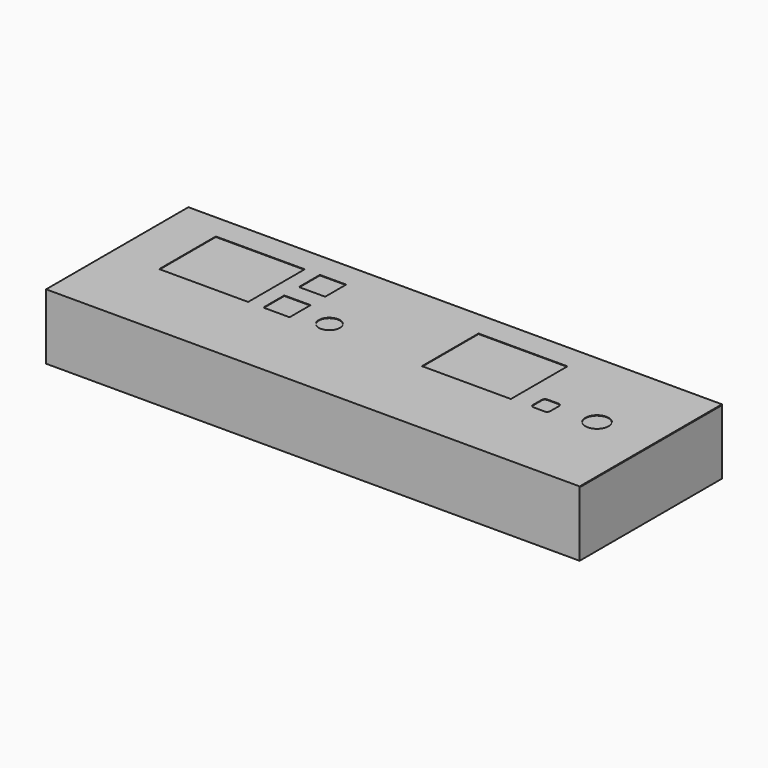
from build123d import *

# Parameters (mm, degrees)
F1_DEPTH = 209.55
F2_W     = 20.6375
F2_H     = 20.6375
F3_DEPTH = 0.4064


# Not quite as in the source:
# - the dataset's text gives a spline's control points without its knots; the knots are read off the source's solid


with BuildPart() as f1:
    # F0 (on Right) → F1 (new body, symmetric)
    with BuildSketch(Plane.YZ):
        Polygon((-139.7, 0), (0, 0), (0, 50.8), (-139.2936, 50.8), (-139.2936, 51.054), (0, 51.054), (0, 51.4604), (-139.7, 51.4604), align=None)
    extrude(amount=F1_DEPTH, both=True)

    # F2 (on face) → F3 (cut, through all)
    with BuildSketch(Plane.XY.offset(51.4604)):
        with BuildLine():
            add(Edge.make_bspline(
                [(120.2687199611, -62.5889714683), (119.8277505611, -63.0292296683), (119.5707533611, -63.6493706683), (119.5707533611, -64.2722294683)],
                knots=[1, 1, 1, 1, 2, 2, 2, 2], degree=3))
            Line((119.5707533611, -64.2722294683), (119.5707533611, -73.0035048683))
            add(Edge.make_bspline(
                [(119.5707533611, -73.0035048683), (119.5707533611, -73.6270748683), (119.8277505611, -74.2471650683), (120.2687199611, -74.6874486683)],
                knots=[0, 0, 0, 0, 1, 1, 1, 1], degree=3))
            add(Edge.make_bspline(
                [(120.2687199611, -74.6874486683), (120.7090289611, -75.1284180683), (121.3291445611, -75.3847548683), (121.9520033611, -75.3847548683)],
                knots=[1, 1, 1, 1, 2, 2, 2, 2], degree=3))
            Line((121.9520033611, -75.3847548683), (130.6832533611, -75.3847548683))
            add(Edge.make_bspline(
                [(130.6832533611, -75.3847548683), (131.3068233611, -75.3847548683), (131.9269389611, -75.1284180683), (132.3671971611, -74.6874486683)],
                knots=[0, 0, 0, 0, 1, 1, 1, 1], degree=3))
            add(Edge.make_bspline(
                [(132.3671971611, -74.6874486683), (132.8081665611, -74.2471650683), (133.0645033611, -73.6270748683), (133.0645033611, -73.0035048683)],
                knots=[1, 1, 1, 1, 2, 2, 2, 2], degree=3))
            Line((133.0645033611, -73.0035048683), (133.0645033611, -64.2722294683))
            add(Edge.make_bspline(
                [(133.0645033611, -64.2722294683), (133.0645033611, -63.6493706683), (132.8081665611, -63.0292296683), (132.3671971611, -62.5889714683)],
                knots=[0, 0, 0, 0, 1, 1, 1, 1], degree=3))
            add(Edge.make_bspline(
                [(132.3671971611, -62.5889714683), (131.9269389611, -62.1480020683), (131.3068233611, -61.8909794683), (130.6832533611, -61.8909794683)],
                knots=[1, 1, 1, 1, 2, 2, 2, 2], degree=3))
            Line((130.6832533611, -61.8909794683), (121.9520033611, -61.8909794683))
            add(Edge.make_bspline(
                [(121.9520033611, -61.8909794683), (121.3291445611, -61.8909794683), (120.7090289611, -62.1480020683), (120.2687199611, -62.5889714683)],
                knots=[0, 0, 0, 0, 1, 1, 1, 1], degree=3))
        make_face()
        Polygon((-172.1320160389, -19.8222294683), (-172.1320160389, -75.3847548683), (-102.2820160389, -75.3847548683), (-102.2821938389, -19.8222294683), align=None)
        Polygon((-90.3757660389, -75.3847548683), (-69.7382660389, -75.3847548683), (-69.7384438389, -54.7472294683), (-90.3759438389, -54.7472294683), align=None)
        with Locations((-80.0571938389, -30.1409794683)):
            Rectangle(F2_W, F2_H)
        Polygon((34.2429839611, -75.3847548683), (104.0926283611, -75.3847548683), (104.0926283611, -19.8222294683), (34.2426283611, -19.8222294683), align=None)
        with BuildLine():
            add(Edge.make_bspline(
                [(-39.2385048389, -61.1578846683), (-40.7817326389, -59.6144790683), (-42.9500798389, -58.7159794683), (-45.1321938389, -58.7159794683)],
                knots=[7, 7, 7, 7, 8, 8, 8, 8], degree=3))
            add(Edge.make_bspline(
                [(-45.1321938389, -58.7159794683), (-47.3139776389, -58.7159794683), (-49.4823248389, -59.6144790683), (-51.0253748389, -61.1578846683)],
                knots=[0, 0, 0, 0, 1, 1, 1, 1], degree=3))
            add(Edge.make_bspline(
                [(-51.0253748389, -61.1578846683), (-52.5684248389, -62.7005790683), (-53.4665688389, -64.8689262683), (-53.4665688389, -67.0503544683), (-53.4665688389, -69.2324684683), (-52.5682470389, -71.4008156683), (-51.0251970389, -72.9442212683)],
                knots=[1, 1, 1, 1, 2, 2, 2, 3, 3, 3, 3], degree=3))
            add(Edge.make_bspline(
                [(-51.0251970389, -72.9442212683), (-49.4821470389, -74.4869664683), (-47.3137998389, -75.3847548683), (-45.1320160389, -75.3847548683), (-42.9499020389, -75.3847548683), (-40.7815548389, -74.4869664683), (-39.2385048389, -72.9442212683)],
                knots=[3, 3, 3, 3, 4, 4, 4, 5, 5, 5, 5], degree=3))
            add(Edge.make_bspline(
                [(-39.2385048389, -72.9442212683), (-37.6957850389, -71.4008156683), (-36.7979966389, -69.2324684683), (-36.7979966389, -67.0503544683), (-36.7979966389, -64.8689262683), (-37.6957850389, -62.7005790683), (-39.2385048389, -61.1578846683)],
                knots=[5, 5, 5, 5, 6, 6, 6, 7, 7, 7, 7], degree=3))
        make_face()
        with BuildLine():
            add(Edge.make_bspline(
                [(170.8727335611, -59.8025914683), (169.1828715611, -58.1123992683), (166.8078445611, -57.1284794683), (164.4179839611, -57.1284794683)],
                knots=[7, 7, 7, 7, 8, 8, 8, 8], degree=3))
            add(Edge.make_bspline(
                [(164.4179839611, -57.1284794683), (162.0281233611, -57.1284794683), (159.6534011611, -58.1123992683), (157.9635899611, -59.8025914683)],
                knots=[0, 0, 0, 0, 1, 1, 1, 1], degree=3))
            add(Edge.make_bspline(
                [(157.9635899611, -59.8025914683), (156.2737533611, -61.4920470683), (155.2898589611, -63.8670740683), (155.2898589611, -66.2566044683), (155.2898589611, -68.6468206683), (156.2737533611, -71.0218730683), (157.9635899611, -72.7113540683)],
                knots=[1, 1, 1, 1, 2, 2, 2, 3, 3, 3, 3], degree=3))
            add(Edge.make_bspline(
                [(157.9635899611, -72.7113540683), (159.6534011611, -74.4015208683), (162.0281233611, -75.3847548683), (164.4179839611, -75.3847548683), (166.8078445611, -75.3847548683), (169.1828715611, -74.4015208683), (170.8727335611, -72.7113540683)],
                knots=[3, 3, 3, 3, 4, 4, 4, 5, 5, 5, 5], degree=3))
            add(Edge.make_bspline(
                [(170.8727335611, -72.7113540683), (172.5625193611, -71.0218730683), (173.5461089611, -68.6468206683), (173.5461089611, -66.2566044683), (173.5461089611, -63.8670740683), (172.5625193611, -61.4920470683), (170.8727335611, -59.8025914683)],
                knots=[5, 5, 5, 5, 6, 6, 6, 7, 7, 7, 7], degree=3))
        make_face()
    extrude(amount=-F3_DEPTH, mode=Mode.SUBTRACT)


solid = f1.part
